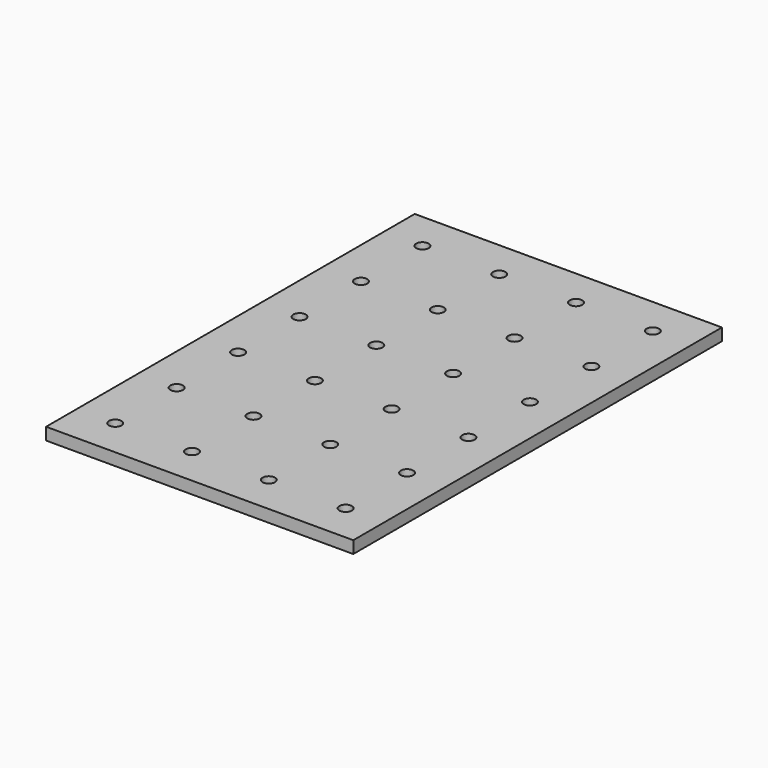
from build123d import *

# Parameters (mm, degrees)
F0_W     = 160
F0_H     = 240
F0_R     = 3.25
F1_DEPTH = 6.35


# Not quite as in the source:
# - a length typed as a fraction of an inch, garbled in the dataset ("3 / 203.2 mm" for 3/8 in), is restored


with BuildPart() as f1:
    # F0 (on Top) → F1 (new body)
    with BuildSketch(Plane.XY):
        Rectangle(F0_W, F0_H)
        with Locations((-60, -100)):
            Circle(F0_R, mode=Mode.SUBTRACT)
        with Locations((-20, -100)):
            Circle(F0_R, mode=Mode.SUBTRACT)
        with Locations((-60, -60)):
            Circle(F0_R, mode=Mode.SUBTRACT)
        with Locations((-60, -20)):
            Circle(F0_R, mode=Mode.SUBTRACT)
        with Locations((-20, -60)):
            Circle(F0_R, mode=Mode.SUBTRACT)
        with Locations((-20, -20)):
            Circle(F0_R, mode=Mode.SUBTRACT)
        with Locations((20, -100)):
            Circle(F0_R, mode=Mode.SUBTRACT)
        with Locations((60, -100)):
            Circle(F0_R, mode=Mode.SUBTRACT)
        with Locations((20, -60)):
            Circle(F0_R, mode=Mode.SUBTRACT)
        with Locations((20, -20)):
            Circle(F0_R, mode=Mode.SUBTRACT)
        with Locations((60, -60)):
            Circle(F0_R, mode=Mode.SUBTRACT)
        with Locations((60, -20)):
            Circle(F0_R, mode=Mode.SUBTRACT)
        with Locations((-60, 20)):
            Circle(F0_R, mode=Mode.SUBTRACT)
        with Locations((-20, 20)):
            Circle(F0_R, mode=Mode.SUBTRACT)
        with Locations((-60, 60)):
            Circle(F0_R, mode=Mode.SUBTRACT)
        with Locations((-60, 100)):
            Circle(F0_R, mode=Mode.SUBTRACT)
        with Locations((-20, 60)):
            Circle(F0_R, mode=Mode.SUBTRACT)
        with Locations((-20, 100)):
            Circle(F0_R, mode=Mode.SUBTRACT)
        with Locations((20, 20)):
            Circle(F0_R, mode=Mode.SUBTRACT)
        with Locations((60, 20)):
            Circle(F0_R, mode=Mode.SUBTRACT)
        with Locations((20, 60)):
            Circle(F0_R, mode=Mode.SUBTRACT)
        with Locations((20, 100)):
            Circle(F0_R, mode=Mode.SUBTRACT)
        with Locations((60, 60)):
            Circle(F0_R, mode=Mode.SUBTRACT)
        with Locations((60, 100)):
            Circle(F0_R, mode=Mode.SUBTRACT)
    extrude(amount=F1_DEPTH)


solid = f1.part
